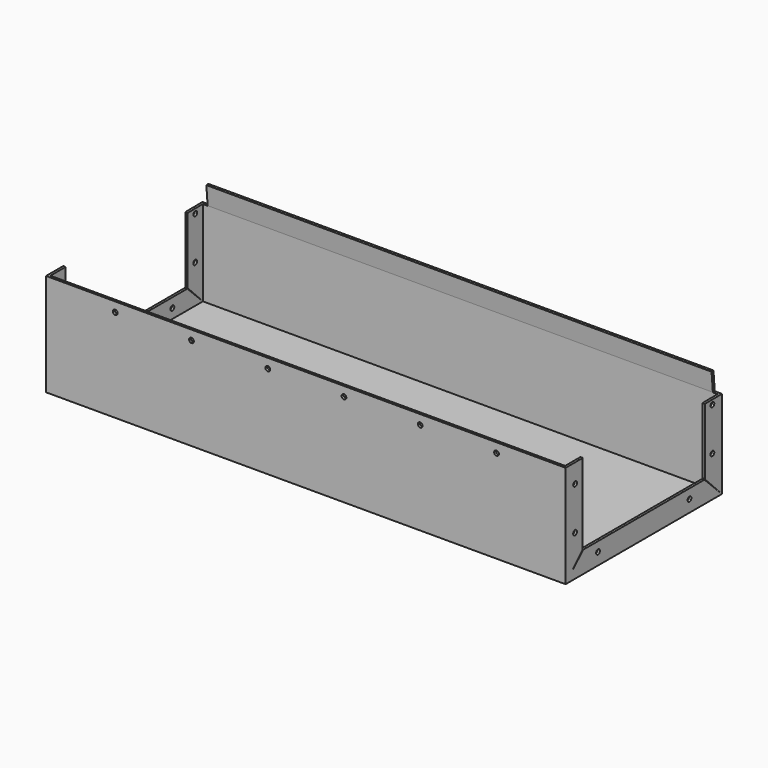
from build123d import *

# Parameters (mm, degrees)
F1_DEPTH  = 342.9
F2_W      = 3.175
F2_H      = 12.7
F3_DEPTH  = 1.5945639921
F5_DEPTH  = 1.5875
F6_DEPTH  = 1.5875
F10_DEPTH = 1.5875
F11_R     = 1.5875
F12_DEPTH = 444.5
F13_R     = 1.5875
F14_DEPTH = 1.5875


# Not quite as in the source:
# - a feature names something its author has since deleted; it is built from what else it names


with BuildPart() as f1:
    # F0 (on Right) → F1 (new body)
    with BuildSketch(Plane.YZ):
        Polygon((0, 68.2625), (0, 0), (130.175, 0), (130.175, 58.7375), (129.0681220671, 71.3891726658), (127.4866629839, 71.2508129242), (128.5875, 58.7375), (128.5875, 1.5875), (1.5875, 1.5875), (1.5875, 68.2625), align=None)
    extrude(amount=F1_DEPTH)

    # F2 (on face) → F3 (cut, through all)
    with BuildSketch(Plane(origin=(0, 134.286004542, 11.7485030676), x_dir=(-1, 0, 0), z_dir=(0, 0.9961946981, 0.0871557427))):
        with Locations((-341.3125, 53.518487267)):
            Rectangle(F2_W, F2_H)
        with Locations((-1.5875, 53.518487267)):
            Rectangle(F2_W, F2_H)
    extrude(amount=-F3_DEPTH, mode=Mode.SUBTRACT)

    # F4 (on face) → F5 (join)
    with BuildSketch(Plane(origin=(0, 0, 0), x_dir=(0, -1, 0), z_dir=(-1, 0, 0))):
        Polygon((-128.5875, 58.5986117467), (-130.175, 58.7375), (-130.175, 0), (-128.5875, 1.6154517363), align=None)
        Polygon((-115.8881750797, 58.5986117466), (-130.175, 58.7375), (-128.5875, 58.5986117467), (-128.5875, 1.6154517363), (-115.8881750797, 14.538378661), align=None)
        Polygon((-115.6359343729, 14.2875), (-128.5595482637, 1.5875), (-1.6154517363, 1.5875), (-14.5390656271, 14.2875), align=None)
        Polygon((-14.2868249203, 14.538378661), (-1.5875, 1.6154517363), (-1.5875, 68.2625), (-14.2868249203, 68.2625), (-14.2868249203, 58.5986117466), align=None)
    extrude(amount=F5_DEPTH)


with BuildPart() as f6:
    # F6 (new): a face of the model
    f6_faces = [f1.part.faces().sort_by_distance(p)[0] for p in [
        (0, 129.2764111618, 0.7047010288),
    ]]
    extrude(f6_faces, amount=F6_DEPTH)


with BuildPart() as f1_1:
    add(f1.part)

    # F7: union F6
    add(f6.part)

    # F9 (on face) + F8 (on face) → F10 (join)
    with BuildSketch(Plane.YZ.offset(342.9)):
        Polygon((1.5875, 68.2625), (1.5875, 1.6154517363), (14.2868249203, 14.538378661), (14.2868249203, 58.5986117466), (14.2868249203, 68.2625), align=None)
        Polygon((115.8881750797, 14.538378661), (128.5875, 1.6154517363), (128.5875, 58.5986117467), (130.175, 58.7375), (115.8881750797, 58.5986117466), align=None)
        Polygon((128.5875, 1.6154517363), (130.175, 0), (130.175, 58.7375), (128.5875, 58.5986117467), align=None)
        Polygon((14.5390656271, 14.2875), (1.6154517363, 1.5875), (128.5595482637, 1.5875), (115.6359343729, 14.2875), align=None)
    with BuildSketch(Plane.YZ.offset(342.9)):
        Polygon((128.5875, 58.5986117467), (128.5875, 1.5875), (1.5875, 1.5875), (1.5875, 68.2625), (0, 68.2625), (0, 0), (130.175, 0), (130.175, 58.7375), align=None)
    extrude(amount=F10_DEPTH)

    # F11 (on face) → F12 (cut, symmetric)
    with BuildSketch(Plane.YZ):
        with Locations((7.9375, 55.5625)):
            Circle(F11_R)
        with Locations((7.9375, 27.0154517363)):
            Circle(F11_R)
        with Locations((26.9875, 7.9654517363)):
            Circle(F11_R)
        with Locations((122.2375, 55.5625)):
            Circle(F11_R)
        with Locations((122.2375, 27.0154517363)):
            Circle(F11_R)
        with Locations((103.1875, 7.9654517363)):
            Circle(F11_R)
    extrude(amount=F12_DEPTH, both=True, mode=Mode.SUBTRACT)

    # F13 (on face) → F14 (cut, through all)
    with BuildSketch(Plane.XZ):
        with Locations((44.45, 61.9125)):
            Circle(F13_R)
        with Locations((95.25, 61.9125)):
            Circle(F13_R)
        with Locations((146.05, 61.9125)):
            Circle(F13_R)
        with Locations((196.85, 61.9125)):
            Circle(F13_R)
        with Locations((247.65, 61.9125)):
            Circle(F13_R)
        with Locations((298.45, 61.9125)):
            Circle(F13_R)
    extrude(amount=-F14_DEPTH, mode=Mode.SUBTRACT)


solid = f1_1.part
